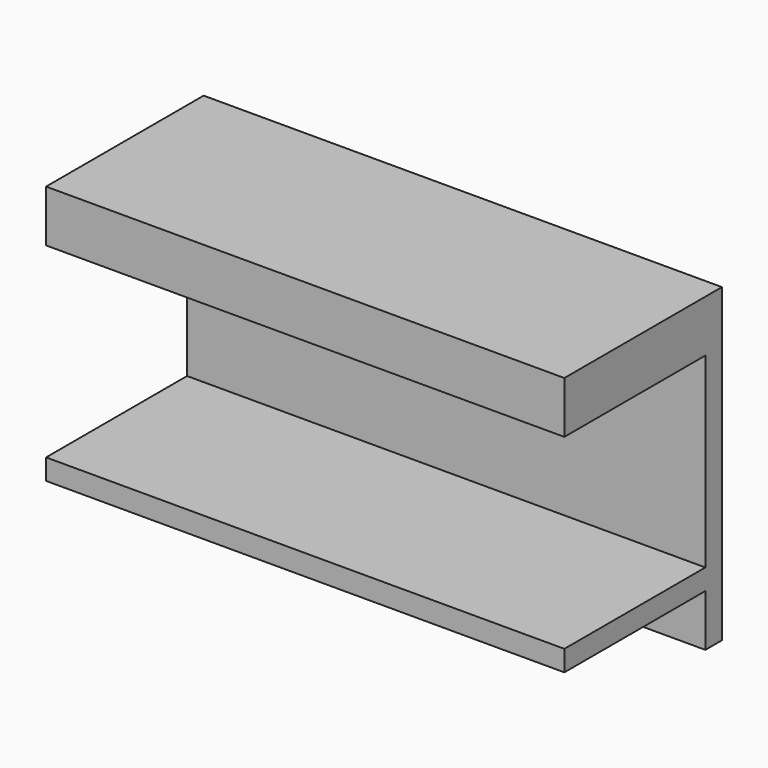
from build123d import *

# Parameters (mm, degrees)
F0_W     = 500
F0_H     = 190
F1_DEPTH = 50
F2_W     = 500
F2_H     = 300
F3_DEPTH = 20
F4_W     = 500
F4_H     = 20
F5_DEPTH = 170


# Not quite as in the source:
# - the program builds the solid bodies; features that only make, move or delete a surface that nothing else refers to are left out


with BuildPart() as f1:
    # F0 (on Top) → F1 (new body)
    with BuildSketch(Plane.XY):
        with Locations((0, -95)):
            Rectangle(F0_W, F0_H)
    extrude(amount=-F1_DEPTH)

    # F2 (on Front) → F3 (join)
    with BuildSketch(Plane.XZ):
        with Locations((0, -150)):
            Rectangle(F2_W, F2_H)
    extrude(amount=F3_DEPTH)

    # F4 (on face) → F5 (join)
    with BuildSketch(Plane.XZ.offset(20)):
        with Locations((0, -240)):
            Rectangle(F4_W, F4_H)
    extrude(amount=F5_DEPTH)


solid = f1.part
